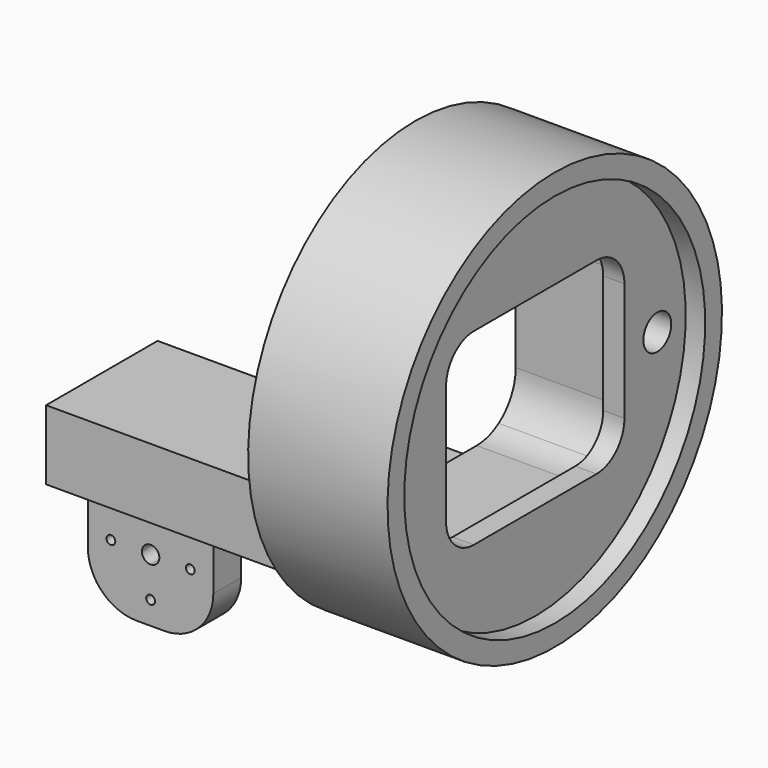
from build123d import *

# Parameters (mm, degrees)
F3_DEPTH = 12.7
F4_DEPTH = 3.175
F5_R     = 8.89
F7_DEPTH = 50.8
F8_DEPTH = 57.15
F2_R     = 3.175
F9_DEPTH = 76.2


with BuildPart() as f1:
    # F0 (on Front) → F1 (revolve)
    with BuildSketch(Plane.XZ):
        Polygon((58.220101, 38.1), (32.820101, 38.1), (32.820101, 0), (54.664101, 0), (54.664101, 34.29), (58.220101, 34.29), align=None)
    revolve(axis=Axis((45.520101, 0, 0), (1, 0, 0)))

    # F0 (on Front) → F3 (join, symmetric)
    with BuildSketch(Plane.XZ):
        Polygon((32.820101, -33.655), (32.820101, -20.955), (-24.329899, -20.955), (-24.329899, -33.655), (-1.469899, -33.655), align=None)
    extrude(amount=F3_DEPTH, both=True)

    # F0 (on Front) → F4 (join, symmetric)
    with BuildSketch(Plane.XZ):
        with BuildLine():
            Line((-1.469899, -56.515), (-1.469899, -45.085))
            Line((-1.469899, -45.085), (-4.860799, -45.085))
            ThreePointArc((-4.860799, -45.085), (-5.660899, -45.8851), (-6.460999, -45.085))
            Line((-6.460999, -45.085), (-11.312399, -45.085))
            ThreePointArc((-11.312399, -45.085), (-11.777367, -46.207532), (-12.899899, -46.6725))
            Line((-12.899899, -46.6725), (-12.899899, -51.5239))
            ThreePointArc((-12.899899, -51.5239), (-12.334143, -51.758244), (-12.099799, -52.324))
            ThreePointArc((-12.099799, -52.324), (-12.334143, -52.889756), (-12.899899, -53.1241))
            Line((-12.899899, -53.1241), (-12.899899, -56.515))
            Line((-12.899899, -56.515), (-1.469899, -56.515))
        make_face()
        with BuildLine():
            Line((-20.938999, -45.085), (-24.329899, -45.085))
            Line((-24.329899, -45.085), (-24.329899, -56.515))
            Line((-24.329899, -56.515), (-12.899899, -56.515))
            Line((-12.899899, -56.515), (-12.899899, -53.1241))
            ThreePointArc((-12.899899, -53.1241), (-13.699999, -52.324), (-12.899899, -51.5239))
            Line((-12.899899, -51.5239), (-12.899899, -46.6725))
            ThreePointArc((-12.899899, -46.6725), (-14.022431, -46.207532), (-14.487399, -45.085))
            Line((-14.487399, -45.085), (-19.338799, -45.085))
            ThreePointArc((-19.338799, -45.085), (-20.138899, -45.8851), (-20.938999, -45.085))
        make_face()
        with BuildLine():
            Line((-1.469899, -45.085), (-1.469899, -33.655))
            Line((-1.469899, -33.655), (-24.329899, -33.655))
            Line((-24.329899, -33.655), (-24.329899, -45.085))
            Line((-24.329899, -45.085), (-20.938999, -45.085))
            ThreePointArc((-20.938999, -45.085), (-20.138899, -44.2849), (-19.338799, -45.085))
            Line((-19.338799, -45.085), (-14.487399, -45.085))
            ThreePointArc((-14.487399, -45.085), (-14.022431, -43.962468), (-12.899899, -43.4975))
            ThreePointArc((-12.899899, -43.4975), (-11.777367, -43.962468), (-11.312399, -45.085))
            Line((-11.312399, -45.085), (-6.460999, -45.085))
            ThreePointArc((-6.460999, -45.085), (-5.660899, -44.2849), (-4.860799, -45.085))
            Line((-4.860799, -45.085), (-1.469899, -45.085))
        make_face()
        with BuildLine():
            ThreePointArc((-12.099799, -37.846), (-12.334143, -38.411756), (-12.899899, -38.6461))
            ThreePointArc((-12.899899, -38.6461), (-13.465656, -37.280244), (-12.099799, -37.846))
        make_face(mode=Mode.SUBTRACT)
    extrude(amount=F4_DEPTH, both=True)

    # F5
    f5_edges = [f1.edges().sort_by_distance(p)[0] for p in [
        (-24.329899, 0, -56.515),
        (-1.469899, 0, -56.515),
    ]]
    fillet(f5_edges, radius=F5_R)

    # F2 (on Right) → F7 (cut)
    with BuildSketch(Plane.YZ):
        with BuildLine():
            Line((13.97, 19.685), (-13.97, 19.685))
            ThreePointArc((-13.97, 19.685), (-20.256179, 17.081179), (-22.86, 10.795))
            Line((-22.86, 10.795), (-22.86, -10.795))
            ThreePointArc((-22.86, -10.795), (-20.256179, -17.081179), (-13.97, -19.685))
            Line((-13.97, -19.685), (13.97, -19.685))
            ThreePointArc((13.97, -19.685), (16.584438, -19.291871), (18.967648, -18.147252))
            ThreePointArc((18.967648, -18.147252), (21.826882, -14.954508), (22.86, -10.795))
            Line((22.86, -10.795), (22.86, 10.795))
            ThreePointArc((22.86, 10.795), (20.256179, 17.081179), (13.97, 19.685))
        make_face()
    extrude(amount=F7_DEPTH, mode=Mode.SUBTRACT)

    # F6 (on Right) → F8 (cut)
    with BuildSketch(Plane.YZ):
        with BuildLine():
            Line((13.97, 17.145), (-13.97, 17.145))
            ThreePointArc((-13.97, 17.145), (-18.460128, 15.285128), (-20.32, 10.795))
            Line((-20.32, 10.795), (-20.32, -10.795))
            ThreePointArc((-20.32, -10.795), (-18.460128, -15.285128), (-13.97, -17.145))
            Line((-13.97, -17.145), (13.97, -17.145))
            ThreePointArc((13.97, -17.145), (18.460128, -15.285128), (20.32, -10.795))
            Line((20.32, -10.795), (20.32, 10.795))
            ThreePointArc((20.32, 10.795), (18.460128, 15.285128), (13.97, 17.145))
        make_face()
    extrude(amount=F8_DEPTH, mode=Mode.SUBTRACT)

    # F2 (on Right) → F9 (cut)
    with BuildSketch(Plane.YZ):
        with Locations((27.813582, 0)):
            Circle(F2_R)
    extrude(amount=F9_DEPTH, mode=Mode.SUBTRACT)


solid = f1.part
